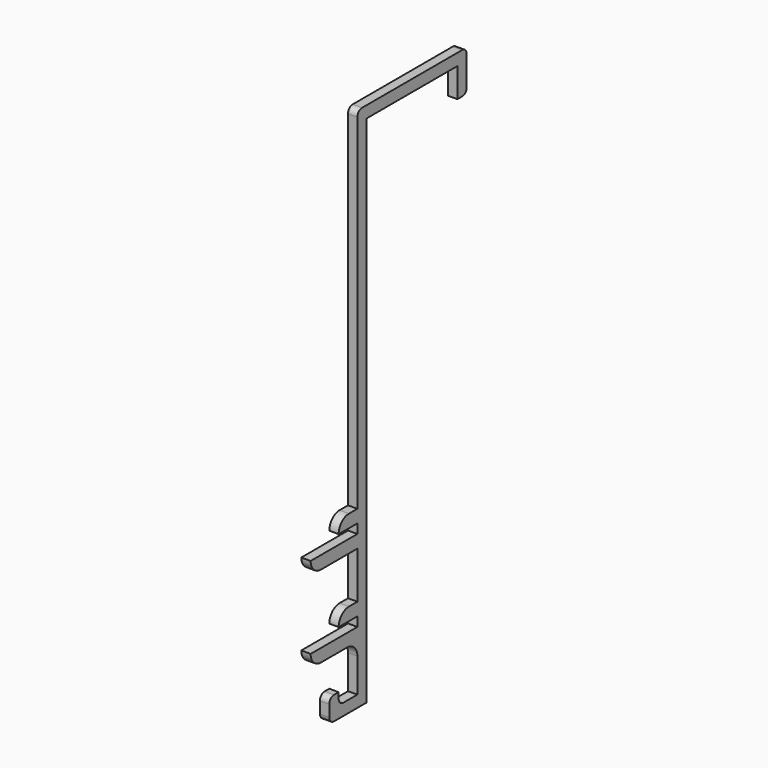
from build123d import *

# Parameters (mm, degrees)
F1_DEPTH = 8
F2_R     = 10.99999
F3_R     = 10.99999
F4_R     = 10.99999
F5_R     = 10.99999
F6_R     = 5
F7_R     = 5


# Not quite as in the source:
# - a fillet or chamfer is up to 0.001 mm smaller than in the source, because OpenCascade refuses the exact size


with BuildPart() as f1:
    # F0 (on Right) → F1 (new body)
    with BuildSketch(Plane.YZ):
        Polygon((115.3961805266, 292.9259983301), (-1.6038194734, 292.9259983301), (-1.6038194734, -7.0740016699), (-21.6038194734, -7.0740016699), (-21.6038194734, -18.0740016699), (-1.6038194734, -18.0740016699), (-1.6038194734, -26.0740016699), (-51.6038194734, -26.0740016699), (-51.6038194734, -37.0740016699), (-1.6038194734, -37.0740016699), (-1.6038194734, -77.0740016699), (-21.6038194734, -77.0740016699), (-21.6038194734, -88.0740016699), (-1.6038194734, -88.0740016699), (-1.6038194734, -96.0740016699), (-51.6038194734, -96.0740016699), (-51.6038194734, -107.0740016699), (-1.6038194734, -107.0740016699), (-1.6038194734, -147.0740016699), (-21.6038194734, -147.0740016699), (-21.6038194734, -137.0740016699), (-31.6038194734, -137.0740016699), (-31.6038194734, -157.0740016699), (8.3961805266, -157.0740016699), (8.3961805266, 282.9259983301), (105.3961805266, 282.9259983301), (105.3961805266, 257.9259983301), (115.3961805266, 257.9259983301), align=None)
    extrude(amount=-F1_DEPTH)

    # F2 (radius 11 in the source; OpenCascade refuses exactly that, so slightly less here)
    f2_edges = [f1.edges().sort_by_distance(p)[0] for p in [
        (-4, -51.603819, -37.074002),
    ]]
    fillet(f2_edges, radius=F2_R)

    # F3 (radius 11 in the source; OpenCascade refuses exactly that, so slightly less here)
    f3_edges = [f1.edges().sort_by_distance(p)[0] for p in [
        (-4, -21.603819, -7.074002),
    ]]
    fillet(f3_edges, radius=F3_R)

    # F4 (radius 11 in the source; OpenCascade refuses exactly that, so slightly less here)
    f4_edges = [f1.edges().sort_by_distance(p)[0] for p in [
        (-4, -21.603819, -77.074002),
    ]]
    fillet(f4_edges, radius=F4_R)

    # F5 (radius 11 in the source; OpenCascade refuses exactly that, so slightly less here)
    f5_edges = [f1.edges().sort_by_distance(p)[0] for p in [
        (-4, -51.603819, -107.074002),
        (-4, -1.603819, -107.074002),
    ]]
    fillet(f5_edges, radius=F5_R)

    # F6
    f6_edges = [f1.edges().sort_by_distance(p)[0] for p in [
        (-4, -31.603819, -137.074002),
        (-4, -31.603819, -157.074002),
        (-4, -21.603819, -147.074002),
    ]]
    fillet(f6_edges, radius=F6_R)

    # F7
    f7_edges = [f1.edges().sort_by_distance(p)[0] for p in [
        (-4, -1.603819, 292.925998),
        (-4, 115.396181, 292.925998),
        (-4, 115.396181, 257.925998),
    ]]
    fillet(f7_edges, radius=F7_R)


solid = f1.part
